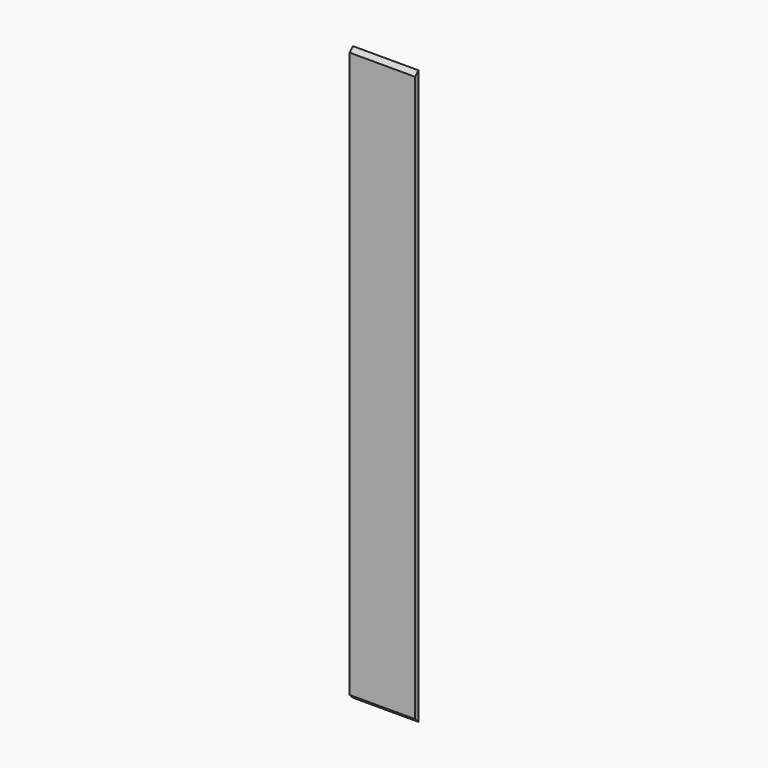
from build123d import *

# Parameters (mm, degrees)
F0_W     = 304.8
F0_H     = 2667
F1_DEPTH = 19.05
F2_SIZE  = 19.04999


# Not quite as in the source:
# - a fillet or chamfer is up to 0.001 mm smaller than in the source, because OpenCascade refuses the exact size


with BuildPart() as f1:
    # F0 (on Front) → F1 (new body)
    with BuildSketch(Plane.XZ):
        with Locations((134.0916193813, 1289.9878754318)):
            Rectangle(F0_W, F0_H)
    extrude(amount=F1_DEPTH)

    # F2 (size 19.05 in the source; OpenCascade refuses exactly that, so slightly less here)
    f2_edges = [f1.edges().sort_by_distance(p)[0] for p in [
        (134.091619, -19.05, 2623.487875),
        (134.091619, -19.05, -43.512125),
    ]]
    chamfer(f2_edges, length=F2_SIZE)


solid = f1.part
